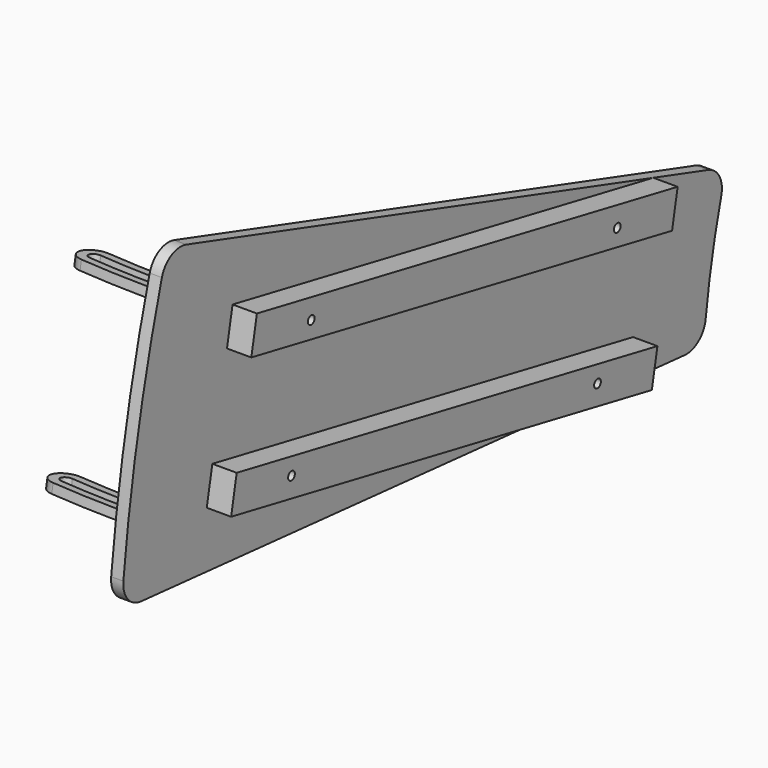
from build123d import *

# Parameters (mm, degrees)
F1_DEPTH  = 12.7
F4_DEPTH  = 25.4
F7_DEPTH  = 9.652
F10_DEPTH = 9.652
F11_R     = 6.35
F12_DEPTH = 25.4
F13_W     = 63.8140652657
F13_H     = 50.8
F14_DEPTH = 101.1923770612
F17_W     = 25.4
F17_H     = 558.8000023101
F18_DEPTH = 38.1
F21_D     = 8.8


# Not quite as in the source:
# - a feature of the source that left no trace in its solid (it failed there, or was rolled back) is left out
# - a pattern or mirror of a feature is missing from the dataset's text; its kind, count and spacing are read off the source's solid


with BuildPart() as f1:
    # F0 (on Right) → F1 (new body)
    with BuildSketch(Plane.YZ):
        with BuildLine():
            ThreePointArc((-756.3314490517, 92.7725130381), (-747.9999137871, 145.3964544769), (-736.0115033336, 197.3095713861))
            ThreePointArc((-736.0115033336, 197.3095713861), (-738.3291312366, 216.1993713631), (-753.1189788115, 228.1766979004))
            Line((-753.1189788115, 228.1766979004), (-1433.4591504296, 436.1775621929))
            ThreePointArc((-1433.4591504296, 436.1775621929), (-1453.0143855451, 434.2043994356), (-1465.30717803, 418.8685641269))
            ThreePointArc((-1465.30717803, 418.8685641269), (-1495.9998275742, 290.7929089539), (-1515.5200833468, 160.5455604257))
            ThreePointArc((-1515.5200833468, 160.5455604257), (-1509.8673096495, 141.7214604148), (-1492.4751711568, 132.5664557537))
            Line((-1492.4751711568, 132.5664557537), (-783.7562532192, 70.5615848078))
            ThreePointArc((-783.7562532192, 70.5615848078), (-765.5565598439, 76.1263941769), (-756.3314490517, 92.7725130381))
        make_face()
        with BuildLine():
            ThreePointArc((-868.3901696878, 137.4879790683), (-863.196533516, 167.7279226013), (-856.9770599652, 197.7736575783))
            ThreePointArc((-856.9770599652, 197.7736575783), (-841.8007632153, 207.3788653824), (-832.1955554113, 192.2025686325))
            ThreePointArc((-832.1955554113, 192.2025686325), (-838.239832524, 163.0031923871), (-843.2871690853, 133.6150782495))
            ThreePointArc((-843.2871690853, 133.6150782495), (-857.775119796, 123.0000283577), (-868.3901696878, 137.4879790683))
        make_face(mode=Mode.SUBTRACT)
        with BuildLine():
            ThreePointArc((-1392.344253737, 220.5256653672), (-1383.7998405062, 268.9834407823), (-1373.5694803277, 317.1135013085))
            ThreePointArc((-1373.5694803277, 317.1135013085), (-1358.3381021148, 326.6311227412), (-1348.8204806822, 311.3997445282))
            ThreePointArc((-1348.8204806822, 311.3997445282), (-1358.8665100466, 264.1368922998), (-1367.2569698858, 216.5522299552))
            ThreePointArc((-1367.2569698858, 216.5522299552), (-1381.7873295174, 205.9953057356), (-1392.344253737, 220.5256653672))
        make_face(mode=Mode.SUBTRACT)
        with BuildLine():
            ThreePointArc((-1348.8204806822, 311.3997445282), (-1358.3381021148, 326.6311227412), (-1373.5694803277, 317.1135013085))
            ThreePointArc((-1373.5694803277, 317.1135013085), (-1383.7998405062, 268.9834407823), (-1392.344253737, 220.5256653672))
            ThreePointArc((-1392.344253737, 220.5256653672), (-1381.7873295174, 205.9953057356), (-1367.2569698858, 216.5522299552))
            ThreePointArc((-1367.2569698858, 216.5522299552), (-1358.8665100466, 264.1368922998), (-1348.8204806822, 311.3997445282))
        make_face()
        with BuildLine():
            ThreePointArc((-832.1955554113, 192.2025686325), (-841.8007632153, 207.3788653824), (-856.9770599652, 197.7736575783))
            ThreePointArc((-856.9770599652, 197.7736575783), (-863.196533516, 167.7279226013), (-868.3901696878, 137.4879790683))
            ThreePointArc((-868.3901696878, 137.4879790683), (-857.775119796, 123.0000283577), (-843.2871690853, 133.6150782495))
            ThreePointArc((-843.2871690853, 133.6150782495), (-838.239832524, 163.0031923871), (-832.1955554113, 192.2025686325))
        make_face()
    extrude(amount=-F1_DEPTH)

    # F3 (on face) → F4 (join, symmetric)
    with BuildSketch(Plane(origin=(0, 0, 0), x_dir=(1, 0, 0), z_dir=(0, -0.1908089954, -0.9816271834))):
        with BuildLine():
            ThreePointArc((-38.1, 829.9252514334), (-33.6098719395, 828.0653794939), (-31.75, 823.5752514334))
            ThreePointArc((-31.75, 823.5752514334), (-33.6098719395, 819.0851233729), (-38.1, 817.2252514334))
            Line((-38.1, 817.2252514334), (-38.1, 810.8752514334))
            ThreePointArc((-38.1, 810.8752514334), (-29.1197438789, 814.5949953123), (-25.4, 823.5752514334))
            ThreePointArc((-25.4, 823.5752514334), (-29.1197438789, 832.5555075545), (-38.1, 836.2752514334))
            Line((-38.1, 836.2752514334), (-38.1, 829.9252514334))
        make_face()
        with BuildLine():
            ThreePointArc((-38.1, 817.2252514334), (-44.45, 823.5752514334), (-38.1, 829.9252514334))
            Line((-38.1, 829.9252514334), (-38.1, 836.2752514334))
            ThreePointArc((-38.1, 836.2752514334), (-50.8, 823.5752514334), (-38.1, 810.8752514334))
            Line((-38.1, 810.8752514334), (-38.1, 817.2252514334))
        make_face()
        with BuildLine():
            Line((-12.7, 836.2752514334), (-38.1, 836.2752514334))
            ThreePointArc((-38.1, 836.2752514334), (-29.1197438789, 832.5555075545), (-25.4, 823.5752514334))
            ThreePointArc((-25.4, 823.5752514334), (-29.1197438789, 814.5949953123), (-38.1, 810.8752514334))
            Line((-38.1, 810.8752514334), (-12.7, 810.8752514334))
            Line((-12.7, 810.8752514334), (-12.7, 836.2752514334))
        make_face()
    extrude(amount=F4_DEPTH, both=True)

    # F9 (on face) → F10 (join)
    with BuildSketch(Plane(origin=(0, -4.8465484826, -24.9333304596), x_dir=(1, 0, 0), z_dir=(0, -0.1908089954, -0.9816271834))):
        with BuildLine():
            Line((-12.7, 810.8752514334), (-12.7, 836.2752514334))
            Line((-12.7, 836.2752514334), (-38.1, 836.2752514334))
            ThreePointArc((-38.1, 836.2752514334), (-50.8, 823.5752514334), (-38.1, 810.8752514334))
            Line((-38.1, 810.8752514334), (-12.7, 810.8752514334))
        make_face()
    f10 = extrude(amount=F10_DEPTH)

    # F10_copies: F10 across plane
    add(f10.mirror(Plane(origin=(0, 0, 0), x_dir=(0, 0.9816271834, -0.1908089954), z_dir=(0, 0.1908089954, 0.9816271834))))

    # F11 (on face) → F12 (cut)
    with BuildSketch(Plane(origin=(0, -6.6882369059, -34.4079960342), x_dir=(1, 0, 0), z_dir=(0, -0.1908089954, -0.9816271834))):
        with Locations((-38.1, 823.5752514334)):
            Circle(F11_R)
    f12 = extrude(amount=-F12_DEPTH, mode=Mode.SUBTRACT)

    # F12_copies: F12 across plane
    add(f12.mirror(Plane(origin=(0, 0, 0), x_dir=(0, 0.9816271834, -0.1908089954), z_dir=(0, 0.1908089954, 0.9816271834))), mode=Mode.SUBTRACT)

    # F13 (on face) → F14 (cut, through all)
    with BuildSketch(Plane(origin=(0, -820.9105196516, 159.5688405843), x_dir=(1, 0, 0), z_dir=(0, -0.9816271834, 0.1908089954))):
        with Locations((-44.6070326328, 0)):
            Rectangle(F13_W, F13_H)
    extrude(amount=-F14_DEPTH, mode=Mode.SUBTRACT)

    # F17 (on face) → F18 (join)
    with BuildSketch(Plane(origin=(0, -9.5404497688, -49.0813591724), x_dir=(1, 0, 0), z_dir=(0, -0.1908089954, -0.9816271834))):
        with Locations((12.7, 1136.5846496688)):
            Rectangle(F17_W, F17_H)
    f18 = extrude(amount=F18_DEPTH)

    # F18_copies: F18 across plane
    add(f18.mirror(Plane(origin=(0, 0, 0), x_dir=(0, 0.9816271834, -0.1908089954), z_dir=(0, 0.1908089954, 0.9816271834))))

    # F21 (through all)
    with Locations(Plane.YZ.offset(25.4)):
        with Locations((-929.1153519156, 111.8383524205), (-1328.0486392687, 189.3831281415), (-1302.2894248929, 321.9027979069), (-903.3561375398, 244.3580221859)):
            Hole(F21_D / 2)


with BuildPart() as f7:
    # F6 (on face) → F7 (new body)
    with BuildSketch(Plane(origin=(0, -19.3861939303, -99.7333218383), x_dir=(1, 0, 0), z_dir=(0, -0.1908089954, -0.9816271834))):
        with BuildLine():
            Line((-12.7, 1458.0670480707), (-12.7, 1474.0815496381))
            ThreePointArc((-12.7, 1474.0815496381), (-65.1564294406, 1474.0147594815), (-117.4371862954, 1469.7247812442))
            ThreePointArc((-117.4371862954, 1469.7247812442), (-131.3697565808, 1451.8919044925), (-113.5368798291, 1437.9593342071))
            ThreePointArc((-113.5368798291, 1437.9593342071), (-63.2019841466, 1442.064066527), (-12.7, 1442.0518993386))
            Line((-12.7, 1442.0518993386), (-12.7, 1458.0670480707))
        make_face()
        with BuildLine():
            ThreePointArc((-38.1, 1464.9252514334), (-31.75, 1458.5752514334), (-38.1, 1452.2252514334))
            ThreePointArc((-38.1, 1452.2252514334), (-76.4781643786, 1451.0526924613), (-114.7131627316, 1447.5393896627))
            ThreePointArc((-114.7131627316, 1447.5393896627), (-121.7897011252, 1453.068187395), (-116.2609033929, 1460.1447257886))
            ThreePointArc((-116.2609033929, 1460.1447257886), (-77.2534808307, 1463.7290044013), (-38.1, 1464.9252514334))
        make_face(mode=Mode.SUBTRACT)
    extrude(amount=-F7_DEPTH)


with BuildPart() as f7_copies_1:
    # F7_copies: instance of F7
    add(f7.part.mirror(Plane(origin=(0, 0, 0), x_dir=(0, 0.9816271834, -0.1908089954), z_dir=(0, 0.1908089954, 0.9816271834))))


solid = Compound([f1.part, f7.part, f7_copies_1.part])
